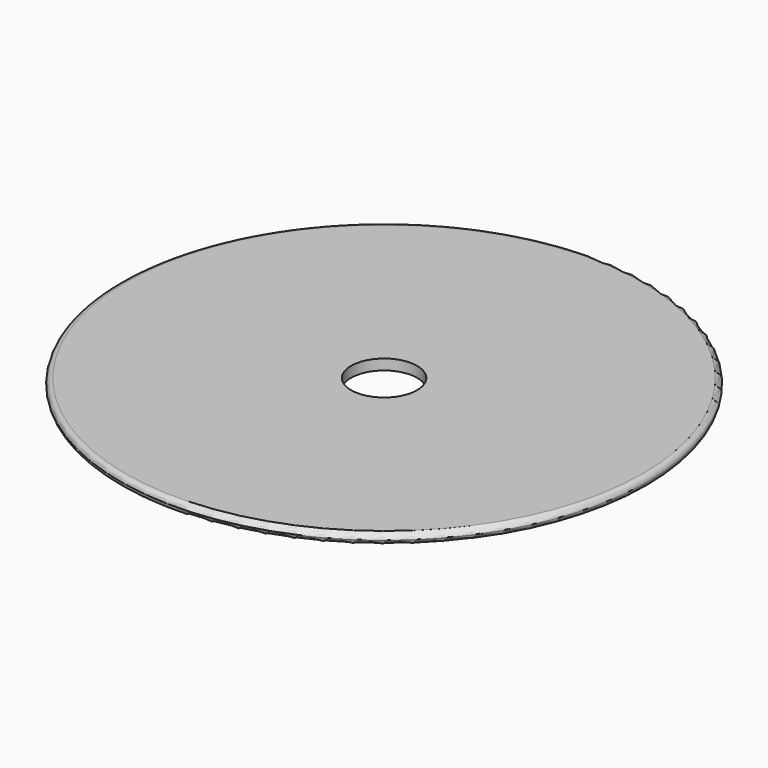
from build123d import *

# Parameters (mm, degrees)
F0_R     = 12.7
F0_R_2   = 1.5875
F1_DEPTH = 0.254
F2_R     = 0.25399


# Not quite as in the source:
# - a fillet or chamfer is up to 0.001 mm smaller than in the source, because OpenCascade refuses the exact size


with BuildPart() as f1:
    # F0 (on Top) → F1 (new body, symmetric)
    with BuildSketch(Plane.XY):
        Circle(F0_R)
        Circle(F0_R_2, mode=Mode.SUBTRACT)
    extrude(amount=F1_DEPTH, both=True)

    # F2 (radius 0.254 in the source; OpenCascade refuses exactly that, so slightly less here)
    f2_edges = [f1.edges().sort_by_distance(p)[0] for p in [
        (-12.7, 0, 0.254),
        (-12.7, 0, -0.254),
    ]]
    fillet(f2_edges, radius=F2_R)


solid = f1.part
